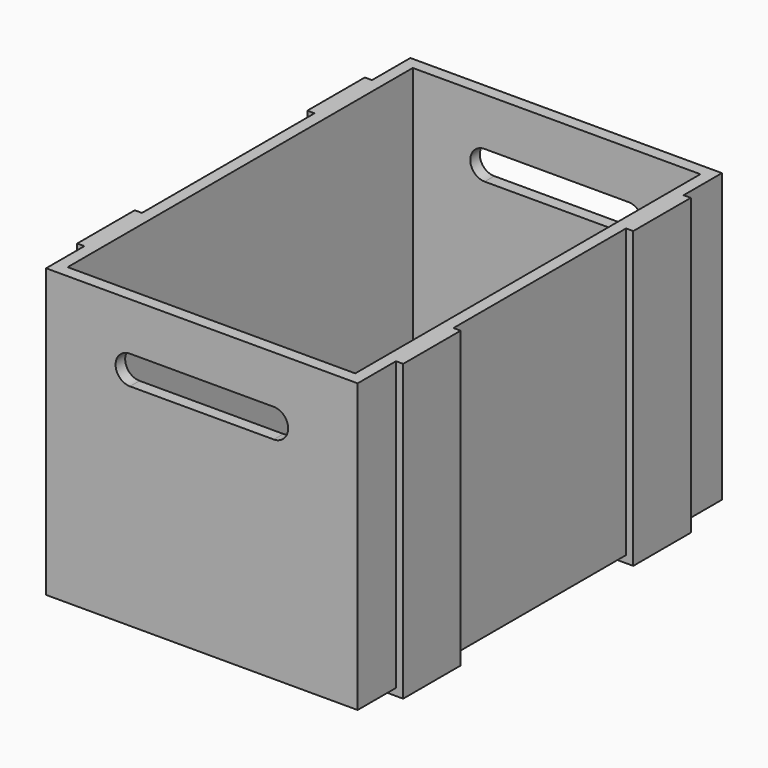
from build123d import *

# Parameters (mm, degrees)
F0_W          = 130
F0_H          = 190
F2_DEPTH      = 120
F3_T          = -5
F5_DEPTH      = 95.001
F5_DEPTH_BACK = 95.001
F6_W          = 130
F6_H          = 30
F7_DEPTH      = 3
F8_W          = 30
F8_H          = 123
F9_DEPTH      = 3


# Not quite as in the source:
# - a pattern or mirror of a feature is missing from the dataset's text; its kind, count and spacing are read off the source's solid


with BuildPart() as f2:
    # F0 (on Top) → F2 (new body, through all)
    with BuildSketch(Plane.XY):
        Rectangle(F0_W, F0_H)
    extrude(amount=F2_DEPTH)

    # F3
    f3_openings = [f2.faces().sort_by_distance(p)[0] for p in [
        (0, 0, 120),
    ]]
    offset(amount=F3_T, openings=f3_openings)

    # F4 (on Front) → F5 (cut, two sides)
    with BuildSketch(Plane.XZ) as f5_sk:
        with BuildLine():
            Line((30, 100), (-30, 100))
            ThreePointArc((-30, 100), (-36, 94), (-30, 88))
            Line((-30, 88), (30, 88))
            ThreePointArc((30, 88), (36, 94), (30, 100))
        make_face()
    extrude(amount=-F5_DEPTH, mode=Mode.SUBTRACT)
    extrude(f5_sk.sketch, amount=F5_DEPTH_BACK, mode=Mode.SUBTRACT)

    # F6 (on face) → F7 (join)
    with BuildSketch(Plane(origin=(0, 0, 0), x_dir=(1, 0, 0), z_dir=(0, 0, -1))):
        with Locations((0, 60)):
            Rectangle(F6_W, F6_H)
        with Locations((0, -60)):
            Rectangle(F6_W, F6_H)
    extrude(amount=F7_DEPTH)

    # F8 (on face) → F9 (join)
    with BuildSketch(Plane.YZ.offset(65)):
        with Locations((-60, 58.5)):
            Rectangle(F8_W, F8_H)
        with Locations((60, 58.5)):
            Rectangle(F8_W, F8_H)
    f9 = extrude(amount=F9_DEPTH)

    # F9_copies: F9 across plane
    add(f9.mirror(Plane(origin=(0, 0, 0), x_dir=(0, 0, -1), z_dir=(-1, 0, 0))))


solid = f2.part
